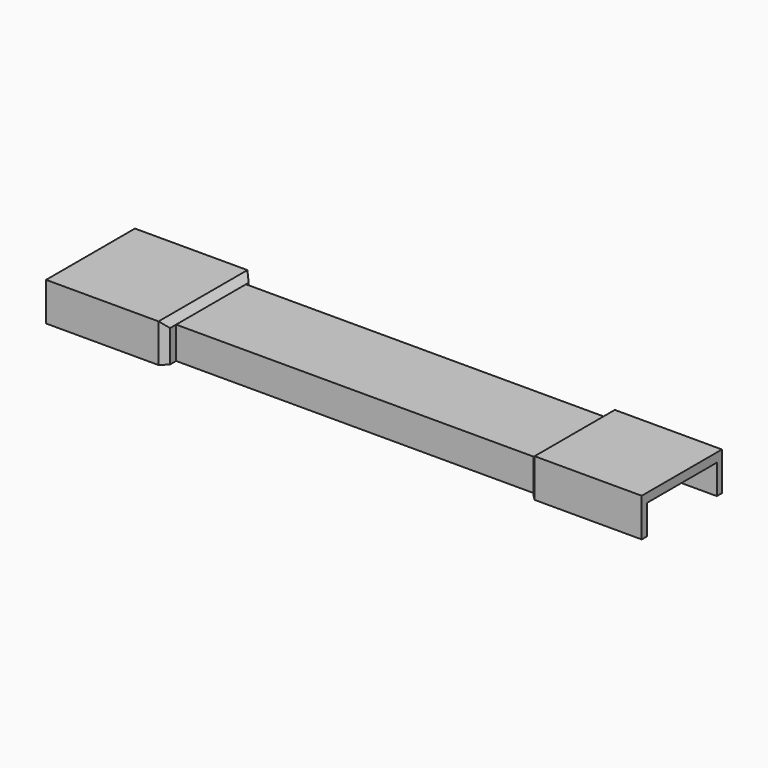
from build123d import *

# Parameters (mm, degrees)
F9_W         = 46.3566482067
F9_H         = 43.3133840561
F10_DEPTH    = 15
F0_W         = 44.2660450935
F0_H         = 39.1066074371
F1_SIZE      = 2.5
F2_SIZE      = 2.5
F3_DEPTH     = 12.5
F4_T         = -2.5
F4_2_T       = -2.5
F4_3_T       = -2.5
F8_T4_DEPTH  = 34.1066074371
F13_T4_DEPTH = 38.3133840561


# Not quite as in the source:
# - a fillet or chamfer that OpenCascade refuses, or shapes differently, is made with other operations: its cross-section is extruded or revolved along the edge and cut away or added
# - the program builds the solid bodies; features that only make, move or delete a surface that nothing else refers to are left out


with BuildPart() as f10:
    # F9 (on Top) → F10 (new body)
    with BuildSketch(Plane.XY):
        with Locations((-79.1433677077, 0)):
            Rectangle(F9_W, F9_H)
    extrude(amount=F10_DEPTH)

    # F2
    f2_edges = [f10.edges().sort_by_distance(p)[0] for p in [
        (-55.965044, -21.656692, 7.5),
        (-55.965044, 0, 15),
        (-55.965044, 21.656692, 7.5),
    ]]
    chamfer(f2_edges, length=F2_SIZE)

    # F4#2
    f4_2_openings = [f10.faces().sort_by_distance(p)[0] for p in [
        (-79.21314, 0, 0),
    ]]
    offset(amount=F4_2_T, openings=f4_2_openings)

    # F13: chamfer of 14 on 1 edges, made by hand


with BuildPart() as f10b:
    # F0 (on Top) → F10, piece 2 (new body)
    with BuildSketch(Plane.XY):
        with Locations((106.1204075813, 0)):
            Rectangle(F0_W, F0_H)
    extrude(amount=F10_DEPTH)

    # F1
    f1_edges = [f10b.edges().sort_by_distance(p)[0] for p in [
        (83.987385, 19.553304, 7.5),
        (83.987385, -19.553304, 7.5),
        (83.987385, 0, 15),
    ]]
    chamfer(f1_edges, length=F1_SIZE)

    # F4#3
    f4_3_openings = [f10b.faces().sort_by_distance(p)[0] for p in [
        (106.197587, 0, 0),
    ]]
    offset(amount=F4_3_T, openings=f4_3_openings)

    # F8: chamfer of 14 on 1 edges, made by hand


with BuildPart() as f3:
    # F11 (on Top) → F3 (new body)
    with BuildSketch(Plane.XY):
        Polygon((85.5761021376, 17.819724977), (-56.4013458788, 17.819724977), (-57.0746399462, -16.2213742733), (85.5761021376, -16.2213742733), align=None)
    extrude(amount=F3_DEPTH)

    # F4
    f4_openings = [f3.faces().sort_by_distance(p)[0] for p in [
        (14.418922, 0.785755, 0),
    ]]
    offset(amount=F4_T, openings=f4_openings)


with BuildPart() as f8_tool2:
    # F8_s3 → F8_t4 (new body)
    with BuildSketch(Plane.XZ.offset(17.0533037186)):
        Polygon((139.7534301281, 0), (125.7534301281, 14), (125.7534301281, 0), align=None)
    extrude(amount=-F8_T4_DEPTH)

    split(bisect_by=Plane.XY.offset(12.5), keep=Keep.BOTTOM)


with BuildPart() as f10b_1:
    add(f10b.part)

    # F8_t1: cut F8_tool2
    add(f8_tool2.part, mode=Mode.SUBTRACT)


with BuildPart() as f13_tool2:
    # F13_s3 → F13_t4 (new body)
    with BuildSketch(Plane.XZ.offset(-19.156692028)):
        Polygon((-113.8216918111, 0), (-99.8216918111, 14), (-99.8216918111, 0), align=None)
    extrude(amount=F13_T4_DEPTH)

    split(bisect_by=Plane.XY.offset(12.5), keep=Keep.BOTTOM)


with BuildPart() as f10_1:
    add(f10.part)

    # F13_t1: cut F13_tool2
    add(f13_tool2.part, mode=Mode.SUBTRACT)


solid = Compound([f3.part, f10b_1.part, f10_1.part])
